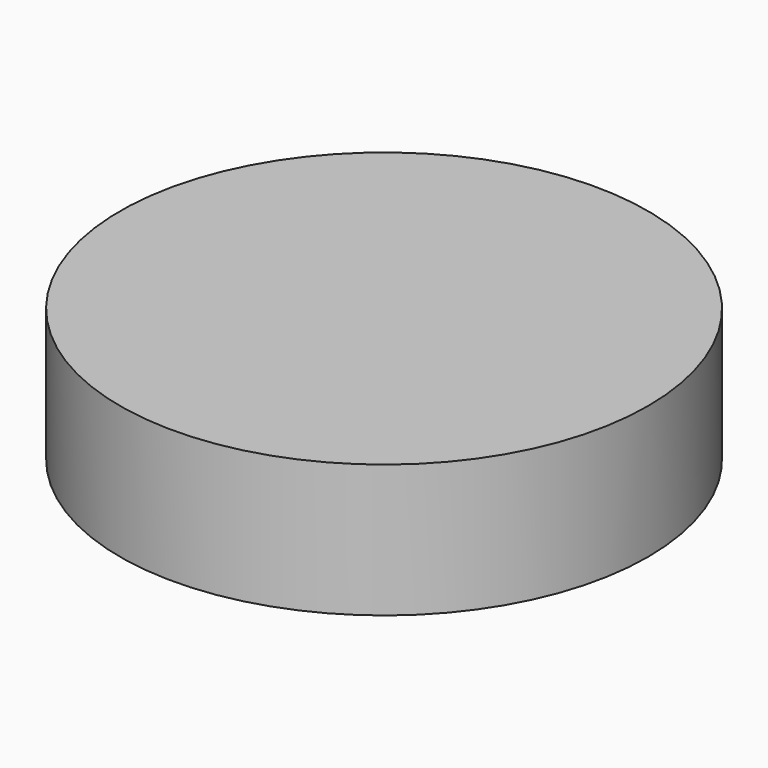
from build123d import *

# Parameters (mm, degrees)
F0_R     = 25.2338276839
F1_DEPTH = 12.7


# Not quite as in the source:
# - a length typed as a fraction of an inch, garbled in the dataset ("3 / 203.2 mm" for 3/8 in), is restored


with BuildPart() as f1:
    # F0 (on Top) → F1 (new body)
    with BuildSketch(Plane.XY):
        Circle(F0_R)
    extrude(amount=F1_DEPTH)


solid = f1.part
